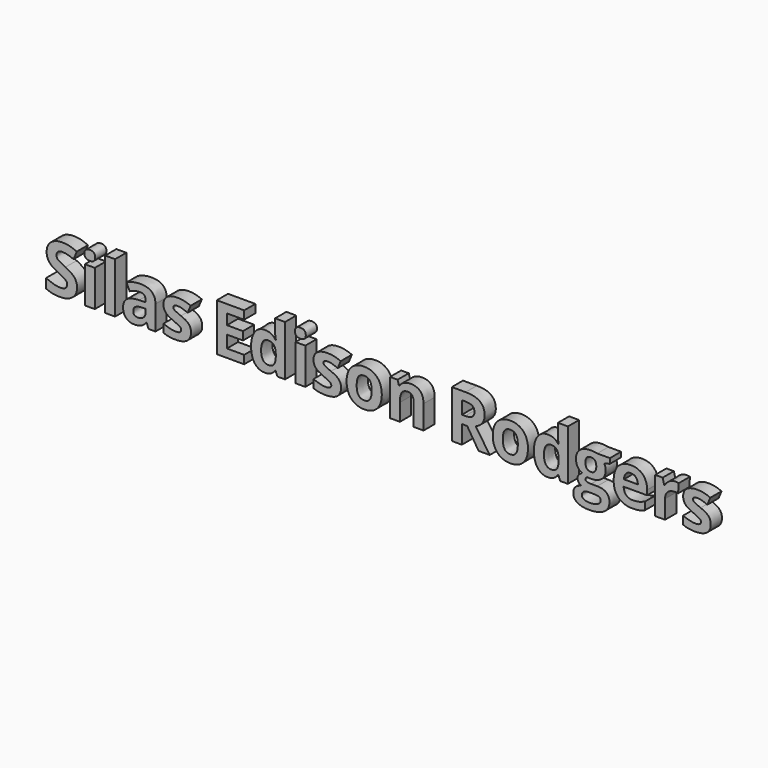
from build123d import *

# Parameters (mm, degrees)
F1_TEXT_SIZE = 15.0902761662
F2_DEPTH     = 3.175


# Not quite as in the source:
# - Text() gives the source's letters only with a copy of the font that has no kerning and outlines rounded to 1/6400 em; it was checked with that copy


with BuildPart() as f2:
    # F1 (on Front) → F2 (new body)
    with BuildSketch(Plane.XZ):
        with Locations((-76.2, -5.4324994198)):
            Text('Silas Edison Rodgers', F1_TEXT_SIZE, font='Open Sans', font_style=FontStyle.BOLD, text_align=(TextAlign.LEFT, TextAlign.BOTTOM))
    extrude(amount=F2_DEPTH)


solid = f2.part
